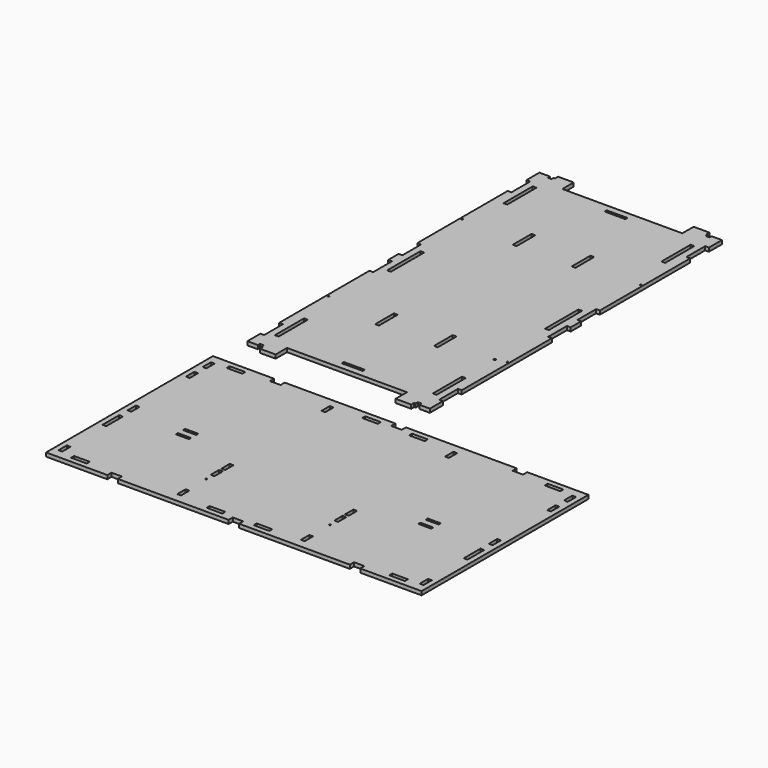
from build123d import *

# Parameters (mm, degrees)
F1_W     = 18.288
F1_H     = 177.8
F1_R     = 3.81
F1_H_2   = 114.3
F1_H_3   = 203.2
F1_R_2   = 5.588
F1_W_2   = 76.2
F1_H_4   = 18.288
F2_DEPTH = 18.288
F1_H_5   = 50.8
F1_W_3   = 63.5
F1_H_6   = 12.7


# Not quite as in the source:
# - a variable given as a bare number and used for a length is read in inches; the dataset says mm whatever the document's units were
# - a feature names something its author has since deleted; it is built from what else it names


with BuildPart() as f2:
    # F1 (on Top) → F2 (new body)
    with BuildSketch(Plane.XY):
        Polygon((-889, 764.9814906911), (-889, 685.8), (-838.2, 685.8), (-838.2, 698.5), (-819.912, 698.5), (-819.912, 685.8), (-812.8, 685.8), (-736.6, 685.8), (-736.6, 736.6), (-152.4, 736.6), (-152.4, 685.8), (-76.2, 685.8), (-69.088, 685.8), (-69.088, 698.5), (-50.8, 698.5), (-50.8, 685.8), (0, 685.8), (0, 764.9814906911), (-18.288, 764.9814906911), (-18.288, 879.2814906911), (0, 879.2814906911), (0, 1428.75), (-18.288, 1428.75), (-18.288, 1543.05), (0, 1543.05), (0, 1606.55), (-18.288, 1606.55), (-18.288, 1720.85), (0, 1720.85), (0, 2270.3185093089), (-18.288, 2270.3185093089), (-18.288, 2384.6185093089), (0, 2384.6185093089), (0, 2463.8), (-50.8, 2463.8), (-50.8, 2451.1), (-69.088, 2451.1), (-69.088, 2463.8), (-76.2, 2463.8), (-152.4, 2463.8), (-152.4, 2413), (-736.6, 2413), (-736.6, 2463.8), (-812.8, 2463.8), (-819.912, 2463.8), (-819.912, 2451.1), (-838.2, 2451.1), (-838.2, 2463.8), (-889, 2463.8), (-889, 2384.6185093089), (-870.712, 2384.6185093089), (-870.712, 2270.3185093089), (-889, 2270.3185093089), (-889, 1720.85), (-870.712, 1720.85), (-870.712, 1606.55), (-889, 1606.55), (-889, 1543.05), (-870.712, 1543.05), (-870.712, 1428.75), (-889, 1428.75), (-889, 879.2814906911), (-870.712, 879.2814906911), (-870.712, 764.9814906911), align=None)
        with Locations((-829.056, 878.8908)):
            Rectangle(F1_W, F1_H, mode=Mode.SUBTRACT)
        Polygon((-393.7, 768.35), (-444.5, 768.35), (-495.3, 768.35), (-495.3, 781.05), (-393.7, 781.05), align=None, mode=Mode.SUBTRACT)
        with Locations((-59.944, 878.8908)):
            Rectangle(F1_W, F1_H, mode=Mode.SUBTRACT)
        with Locations((-879.856, 1168.4)):
            Circle(F1_R, mode=Mode.SUBTRACT)
        with Locations((-587.756, 1155.7)):
            Rectangle(F1_W, F1_H_2, mode=Mode.SUBTRACT)
        with Locations((-829.056, 1574.8)):
            Rectangle(F1_W, F1_H_3, mode=Mode.SUBTRACT)
        with Locations((-301.244, 1155.7)):
            Rectangle(F1_W, F1_H_2, mode=Mode.SUBTRACT)
        with Locations((-59.944, 1155.7)):
            Circle(F1_R_2, mode=Mode.SUBTRACT)
        with Locations((-9.144, 1168.4)):
            Circle(F1_R, mode=Mode.SUBTRACT)
        with Locations((-59.944, 1574.8)):
            Rectangle(F1_W, F1_H_3, mode=Mode.SUBTRACT)
        with Locations((-879.856, 1981.2)):
            Circle(F1_R, mode=Mode.SUBTRACT)
        with Locations((-587.756, 1993.9)):
            Rectangle(F1_W, F1_H_2, mode=Mode.SUBTRACT)
        with Locations((-829.056, 2270.7092)):
            Rectangle(F1_W, F1_H, mode=Mode.SUBTRACT)
        with Locations((-301.244, 1993.9)):
            Rectangle(F1_W, F1_H_2, mode=Mode.SUBTRACT)
        with Locations((-9.144, 1981.2)):
            Circle(F1_R, mode=Mode.SUBTRACT)
        Polygon((-444.5, 2381.25), (-393.7, 2381.25), (-393.7, 2368.55), (-495.3, 2368.55), (-495.3, 2381.25), align=None, mode=Mode.SUBTRACT)
        with Locations((-59.944, 2270.7092)):
            Rectangle(F1_W, F1_H, mode=Mode.SUBTRACT)
        with Locations((-774.7, 2472.944)):
            Rectangle(F1_W_2, F1_H_4)
        with Locations((-114.3, 2472.944)):
            Rectangle(F1_W_2, F1_H_4)
        with Locations((-114.3, 676.656)):
            Rectangle(F1_W_2, F1_H_4)
        with Locations((-774.7, 676.656)):
            Rectangle(F1_W_2, F1_H_4)
    extrude(amount=F2_DEPTH)


with BuildPart() as f2b:
    # F1 (on Top) → F2, piece 2 (new body)
    with BuildSketch(Plane.XY):
        Polygon((914.4, -508), (914.4, 508), (615.95, 508), (615.95, 482.6), (565.15, 482.6), (565.15, 508), (25.4, 508), (25.4, 482.6), (-25.4, 482.6), (-25.4, 508), (-565.15, 508), (-565.15, 482.6), (-615.95, 482.6), (-615.95, 508), (-914.4, 508), (-914.4, -508), (-615.95, -508), (-615.95, -482.6), (-565.15, -482.6), (-565.15, -508), (-25.4, -508), (-25.4, -482.6), (25.4, -482.6), (25.4, -508), (565.15, -508), (565.15, -482.6), (615.95, -482.6), (615.95, -508), align=None)
        with Locations((-879.856, -438.912)):
            Rectangle(F1_W, F1_H_5, mode=Mode.SUBTRACT)
        with Locations((-774.7, -473.456)):
            Rectangle(F1_W_2, F1_H_4, mode=Mode.SUBTRACT)
        Polygon((-889, -196.088), (-889, -145.288), (-889, -94.488), (-870.712, -94.488), (-870.712, -145.288), (-870.712, -196.088), align=None, mode=Mode.SUBTRACT)
        with Locations((-879.856, -18.288)):
            Rectangle(F1_W, F1_H_5, mode=Mode.SUBTRACT)
        with Locations((-590.55, -76.962)):
            Rectangle(F1_W_3, F1_H_6, mode=Mode.SUBTRACT)
        with Locations((-590.55, -32.512)):
            Rectangle(F1_W_3, F1_H_6, mode=Mode.SUBTRACT)
        with Locations((-301.244, -438.912)):
            Rectangle(F1_W, F1_H_5, mode=Mode.SUBTRACT)
        with Locations((-301.244, -299.212)):
            Circle(F1_R, mode=Mode.SUBTRACT)
        with Locations((-301.244, -235.712)):
            Rectangle(F1_W, F1_H_5, mode=Mode.SUBTRACT)
        with Locations((-301.244, -170.688)):
            Rectangle(F1_W, F1_H_5, mode=Mode.SUBTRACT)
        with Locations((-114.3, -473.456)):
            Rectangle(F1_W_2, F1_H_4, mode=Mode.SUBTRACT)
        with Locations((-879.856, 337.312)):
            Rectangle(F1_W, F1_H_5, mode=Mode.SUBTRACT)
        with Locations((-879.856, 438.912)):
            Rectangle(F1_W, F1_H_5, mode=Mode.SUBTRACT)
        with Locations((-774.7, 473.456)):
            Rectangle(F1_W_2, F1_H_4, mode=Mode.SUBTRACT)
        with Locations((-301.244, 438.912)):
            Rectangle(F1_W, F1_H_5, mode=Mode.SUBTRACT)
        with Locations((-114.3, 473.456)):
            Rectangle(F1_W_2, F1_H_4, mode=Mode.SUBTRACT)
        with Locations((114.3, -473.456)):
            Rectangle(F1_W_2, F1_H_4, mode=Mode.SUBTRACT)
        with Locations((301.244, -438.912)):
            Rectangle(F1_W, F1_H_5, mode=Mode.SUBTRACT)
        with Locations((301.244, -299.212)):
            Circle(F1_R, mode=Mode.SUBTRACT)
        with Locations((301.244, -235.712)):
            Rectangle(F1_W, F1_H_5, mode=Mode.SUBTRACT)
        with Locations((301.244, -170.688)):
            Rectangle(F1_W, F1_H_5, mode=Mode.SUBTRACT)
        with Locations((774.7, -473.456)):
            Rectangle(F1_W_2, F1_H_4, mode=Mode.SUBTRACT)
        with Locations((879.856, -438.912)):
            Rectangle(F1_W, F1_H_5, mode=Mode.SUBTRACT)
        Polygon((870.712, -94.488), (889, -94.488), (889, -145.288), (889, -196.088), (870.712, -196.088), (870.712, -145.288), align=None, mode=Mode.SUBTRACT)
        with Locations((590.55, -76.962)):
            Rectangle(F1_W_3, F1_H_6, mode=Mode.SUBTRACT)
        with Locations((590.55, -32.512)):
            Rectangle(F1_W_3, F1_H_6, mode=Mode.SUBTRACT)
        with Locations((879.856, -18.288)):
            Rectangle(F1_W, F1_H_5, mode=Mode.SUBTRACT)
        with Locations((114.3, 473.456)):
            Rectangle(F1_W_2, F1_H_4, mode=Mode.SUBTRACT)
        with Locations((301.244, 438.912)):
            Rectangle(F1_W, F1_H_5, mode=Mode.SUBTRACT)
        with Locations((879.856, 337.312)):
            Rectangle(F1_W, F1_H_5, mode=Mode.SUBTRACT)
        with Locations((774.7, 473.456)):
            Rectangle(F1_W_2, F1_H_4, mode=Mode.SUBTRACT)
        with Locations((879.856, 438.912)):
            Rectangle(F1_W, F1_H_5, mode=Mode.SUBTRACT)
    extrude(amount=F2_DEPTH)


solid = Compound([f2.part, f2b.part])
